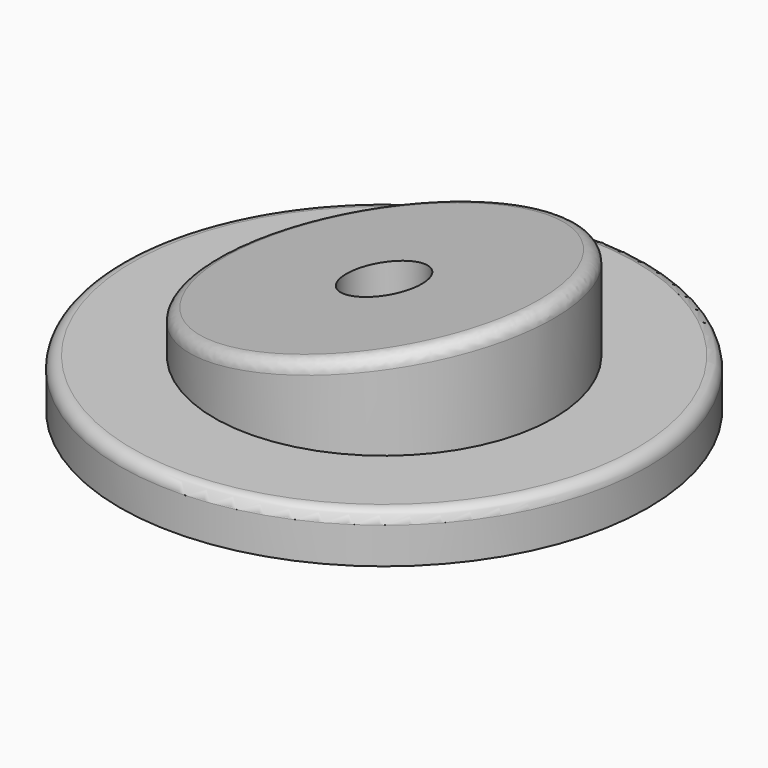
from build123d import *

# Parameters (mm, degrees)
F0_R          = 11.1125
F0_R_2        = 7.14375
F1_DEPTH      = 2.032
F0_R_3        = 1.5875
F2_DEPTH      = 6.35
F4_DEPTH      = 11.1135
F4_DEPTH_BACK = 11.1135
F5_R          = 3.96875
F5_R_2        = 1.5875
F6_DEPTH      = 3.048
F7_R          = 0.508


with BuildPart() as f1:
    # F0 (on Top) → F1 (new body)
    with BuildSketch(Plane.XY):
        Circle(F0_R)
        Circle(F0_R_2, mode=Mode.SUBTRACT)
    extrude(amount=F1_DEPTH)

    # F0 (on Top) → F2 (join)
    with BuildSketch(Plane.XY):
        Circle(F0_R_2)
        Circle(F0_R_3, mode=Mode.SUBTRACT)
    extrude(amount=F2_DEPTH)

    # F3 (on Front) → F4 (cut, two sides)
    with BuildSketch(Plane.XZ) as f4_sk:
        Polygon((7.14375, 6.35), (-7.14375, 6.35), (-7.14375, 3.3864264842), align=None)
    extrude(amount=-F4_DEPTH, mode=Mode.SUBTRACT)
    extrude(f4_sk.sketch, amount=F4_DEPTH_BACK, mode=Mode.SUBTRACT)

    # F5 (on face) → F6 (cut)
    with BuildSketch(Plane(origin=(0, 0, 0), x_dir=(1, 0, 0), z_dir=(0, 0, -1))):
        Circle(F5_R)
        Circle(F5_R_2, mode=Mode.SUBTRACT)
    extrude(amount=-F6_DEPTH, mode=Mode.SUBTRACT)

    # F7
    f7_edges = [f1.edges().sort_by_distance(p)[0] for p in [
        (0, -7.14375, 4.868213),
        (0, 7.14375, 4.868213),
        (-11.1125, 0, 2.032),
    ]]
    fillet(f7_edges, radius=F7_R)


solid = f1.part
